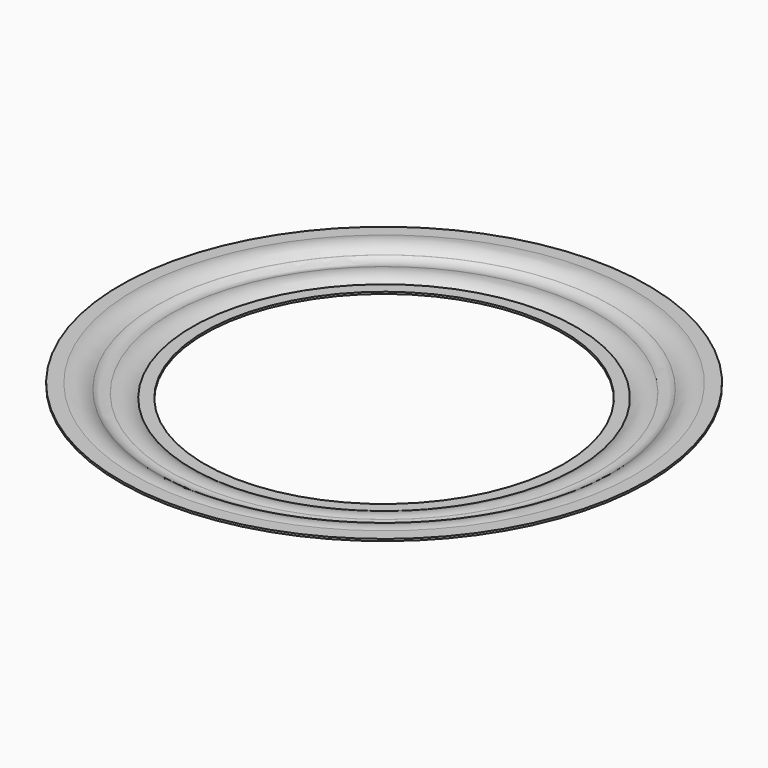
from build123d import *


# Not quite as in the source:
# - ends of sketch curves that miss each other by under 0.0002 mm in the source are joined


with BuildPart() as f1:
    # F0 (on Front) → F1 (revolve)
    with BuildSketch(Plane.XZ):
        with BuildLine():
            Line((0.96, 0), (0.01, 0))
            Line((0.01, 0), (0.01, -0.15))
            Line((0.01, -0.15), (0.96, -0.15))
            ThreePointArc((0.96, -0.15), (1.7476920727, 0.2023696464), (2.61, 0.1700006461))
            ThreePointArc((2.61, 0.1700006461), (2.6139996854, 0.1689036293), (2.6179969666, 0.1677978844))
            ThreePointArc((2.6179969666, 0.1677978844), (3.1597730322, 0.1590424375), (3.64, 0.4100006461))
            ThreePointArc((3.64, 0.4100006461), (3.6431863407, 0.4128835368), (3.646379193, 0.4157592141))
            ThreePointArc((3.646379193, 0.4157592141), (4.4496112836, 0.8443127993), (5.36, 0.8500006461))
            Line((5.36, 0.8500006461), (6.41, 0.8500006461))
            Line((6.41, 0.8500006461), (6.41, 1))
            Line((6.41, 1), (5.36, 1))
            ThreePointArc((5.36, 1), (4.4496112836, 0.9943121532), (3.646379193, 0.565758568))
            ThreePointArc((3.646379193, 0.565758568), (3.6431863407, 0.5628828907), (3.64, 0.56))
            ThreePointArc((3.64, 0.56), (3.1597730322, 0.3090417914), (2.6179969666, 0.3177972383))
            ThreePointArc((2.6179969666, 0.3177972383), (2.6139996854, 0.3189029832), (2.61, 0.32))
            ThreePointArc((2.61, 0.32), (1.7476920727, 0.3523690002), (0.96, 0))
        make_face()
    revolve(axis=Axis((-13.59, 0, 6.1745331623), (0, 0, 1)))


solid = f1.part
